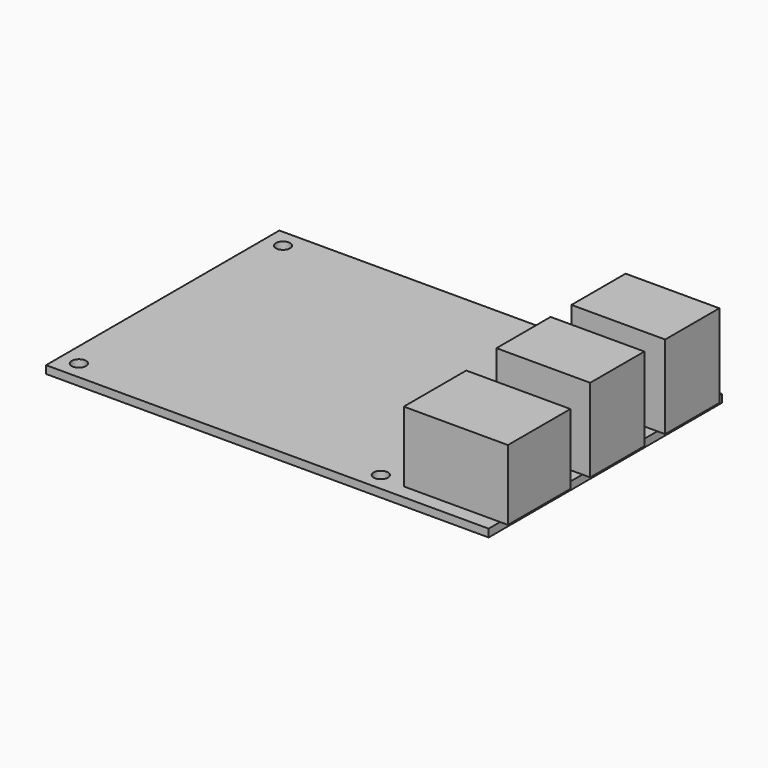
from build123d import *

# Parameters (mm, degrees)
F0_W     = 85
F0_H     = 56
F0_R     = 1.375
F1_DEPTH = 1.5
F3_W     = 18
F3_H     = 13
F4_DEPTH = 16
F3_W_2   = 20
F3_H_2   = 15
F5_DEPTH = 13.5


# Not quite as in the source:
# - a feature names something its author has since deleted; it is built from what else it names


with BuildPart() as f1:
    # F0 (on Top) → F1 (new body)
    with BuildSketch(Plane.XY):
        with Locations((42.5, 28)):
            Rectangle(F0_W, F0_H)
        with Locations((3.5, 3.5)):
            Circle(F0_R, mode=Mode.SUBTRACT)
        with Locations((61.5, 3.5)):
            Circle(F0_R, mode=Mode.SUBTRACT)
        with Locations((3.5, 52.5)):
            Circle(F0_R, mode=Mode.SUBTRACT)
        with Locations((61.5, 52.5)):
            Circle(F0_R, mode=Mode.SUBTRACT)
    extrude(amount=F1_DEPTH)

    # F3 (on offset) → F4 (join)
    with BuildSketch(Plane.XY.offset(1.5)):
        with Locations((77.5, 47)):
            Rectangle(F3_W, F3_H)
        with Locations((77.5, 29)):
            Rectangle(F3_W, F3_H)
    extrude(amount=F4_DEPTH)

    # F3 (on offset) → F5 (join)
    with BuildSketch(Plane.XY.offset(1.5)):
        with Locations((76.5, 10.25)):
            Rectangle(F3_W_2, F3_H_2)
    extrude(amount=F5_DEPTH)


solid = f1.part
